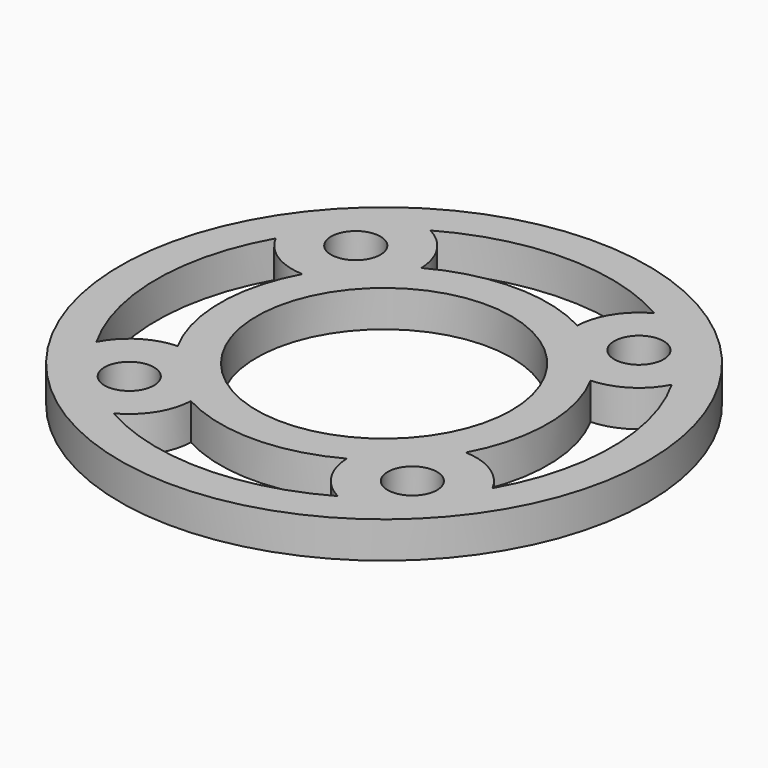
from build123d import *

# Parameters (mm, degrees)
F0_R            = 23.01875
F0_R_2          = 2.15265
F0_R_3          = 11.1125
F1_DEPTH        = 3.175
F3_DEPTH        = 3.175
F3_COPIES_COUNT = 4


# Not quite as in the source:
# - a pattern or mirror of a feature is missing from the dataset's text; its kind, count and spacing are read off the source's solid


with BuildPart() as f1:
    # F0 (on Top) → F1 (new body)
    with BuildSketch(Plane.XY):
        Circle(F0_R)
        with Locations((-12.3478521665, -12.3478521665)):
            Circle(F0_R_2, mode=Mode.SUBTRACT)
        with Locations((12.3478521665, -12.3478521665)):
            Circle(F0_R_2, mode=Mode.SUBTRACT)
        with Locations((-12.3478521665, 12.3478521665)):
            Circle(F0_R_2, mode=Mode.SUBTRACT)
        Circle(F0_R_3, mode=Mode.SUBTRACT)
        with Locations((12.3478521665, 12.3478521665)):
            Circle(F0_R_2, mode=Mode.SUBTRACT)
    extrude(amount=F1_DEPTH)

    # F2 (on face) → F3 (cut, through all)
    with BuildSketch(Plane.XY.offset(3.175)):
        with BuildLine():
            ThreePointArc((-9.7719120136, 17.2709047146), (-7.6525973796, 15.318794197), (-6.7959542154, 12.5677230456))
            ThreePointArc((-6.7959542154, 12.5677230456), (0, 14.2875), (6.7959542154, 12.5677230456))
            ThreePointArc((6.7959542154, 12.5677230456), (7.6525973796, 15.318794197), (9.7719120136, 17.2709047146))
            ThreePointArc((9.7719120136, 17.2709047146), (0, 19.84375), (-9.7719120136, 17.2709047146))
        make_face()
    f3 = extrude(amount=-F3_DEPTH, mode=Mode.SUBTRACT)

    # F3_copies: F3 ×4 about axis
    f3_copies_axis = Axis((0, 0, 0), (0, 0, 1))
    for i in range(1, F3_COPIES_COUNT):
        add(f3.rotate(f3_copies_axis, i * 360 / F3_COPIES_COUNT), mode=Mode.SUBTRACT)


solid = f1.part
